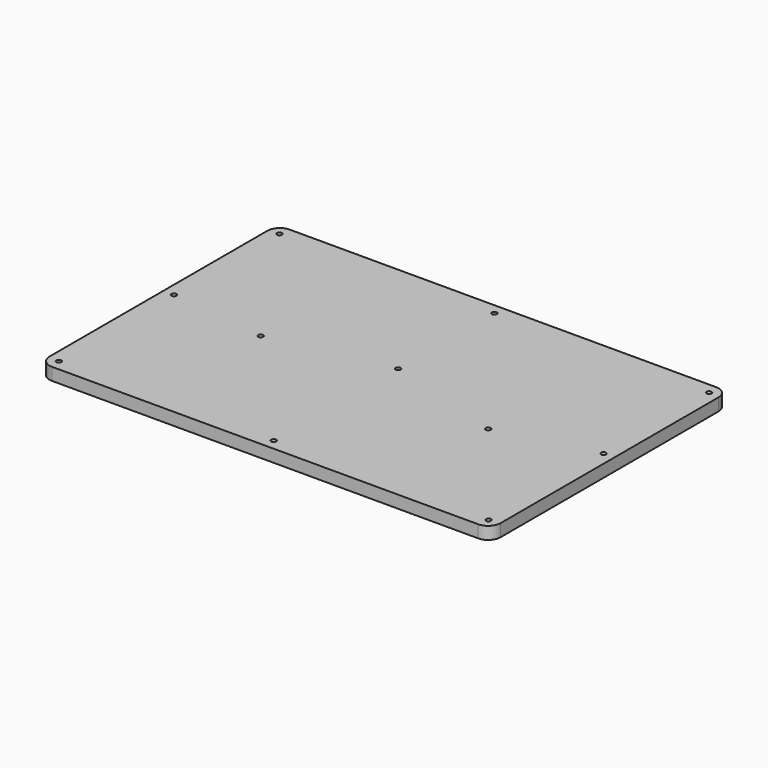
from build123d import *

# Parameters (mm, degrees)
F0_W     = 181.450293
F0_H     = 119.538183
F0_W_2   = 0.80067
F0_H_2   = 5.7989
F0_W_3   = 0.8006
F0_H_3   = 5.8003
F0_W_4   = 0.8007
F0_W_5   = 0.8008
F0_H_4   = 5.801
F0_H_5   = 5.8002
F0_H_6   = 5.7987
F0_W_6   = 0.801
F0_W_7   = 0.8
F0_W_8   = 0.875
F0_H_7   = 2.8002
F1_DEPTH = 5
F3_R     = 5
F2_R     = 1
F4_DEPTH = 5
F5_R     = 1.8
F5_R_2   = 1
F6_DEPTH = 2.5


# Not quite as in the source:
# - a feature names something its author has since deleted; it is built from what else it names


with BuildPart() as f1:
    # F0 (on Top) → F1 (new body)
    with BuildSketch(Plane.XY):
        with Locations((5e-07, 5e-07)):
            Rectangle(F0_W, F0_H)
        Polygon((-67.5631612539, -51.819168), (-73.900653, -51.819168), (-76.699453, -51.819168), (-85.1413756609, -51.819168), (-85.1413756609, -19.618408), (-76.699453, -19.618408), (-73.900653, -19.618408), (-67.5631612539, -19.618408), align=None, mode=Mode.SUBTRACT)
        Polygon((-49.349453, -43.381508), (-49.349453, -46.480608), (-49.349453, -48.281108), (-64.950353, -48.281108), (-64.950353, -46.480608), (-64.950353, -43.381508), (-64.950353, -37.581308), (-64.950353, -34.480708), (-64.950353, -32.681608), (-49.349453, -32.681608), (-49.349453, -34.480708), (-49.349453, -37.581308), align=None, mode=Mode.SUBTRACT)
        Polygon((-30.299453, -33.856508), (-30.299453, -36.955608), (-30.299453, -38.756108), (-45.900353, -38.756108), (-45.900353, -36.955608), (-45.900353, -33.856508), (-45.900353, -28.056308), (-45.900353, -24.955708), (-45.900353, -23.156508), (-30.299453, -23.156508), (-30.299453, -24.955708), (-30.299453, -28.056308), align=None, mode=Mode.SUBTRACT)
        Polygon((-11.249453, -38.619008), (-11.249453, -41.719508), (-11.249453, -43.518608), (-26.850353, -43.518608), (-26.850353, -41.719508), (-26.850353, -38.619008), (-26.850353, -32.818808), (-26.850353, -29.719608), (-26.850353, -27.919108), (-11.249453, -27.919108), (-11.249453, -29.719608), (-11.249453, -32.818808), align=None, mode=Mode.SUBTRACT)
        Polygon((-49.349453, -24.331508), (-49.349453, -27.430608), (-49.349453, -29.231108), (-64.950353, -29.231108), (-64.950353, -27.430608), (-64.950353, -24.331508), (-64.950353, -18.531208), (-64.950353, -15.430608), (-64.950353, -13.631508), (-49.349453, -13.631508), (-49.349453, -15.430608), (-49.349453, -18.531208), align=None, mode=Mode.SUBTRACT)
        Polygon((-68.399553, -10.044008), (-68.399553, -13.144608), (-68.399553, -14.943708), (-84.000333, -14.943708), (-84.000333, -13.144608), (-84.000333, -10.044008), (-84.000333, -4.243708), (-84.000333, -1.144508), (-84.000333, 0.655992), (-68.399553, 0.655992), (-68.399553, -1.144508), (-68.399553, -4.243708), align=None, mode=Mode.SUBTRACT)
        Polygon((-49.349453, -5.281508), (-49.349453, -8.380708), (-49.349453, -10.181208), (-64.950353, -10.181208), (-64.950353, -8.380708), (-64.950353, -5.281508), (-64.950353, 0.518792), (-64.950353, 3.619392), (-64.950353, 5.418492), (-49.349453, 5.418492), (-49.349453, 3.619392), (-49.349453, 0.518792), align=None, mode=Mode.SUBTRACT)
        Polygon((-11.249453, -19.569008), (-11.249453, -22.669608), (-11.249453, -24.468708), (-26.850353, -24.468708), (-26.850353, -22.669608), (-26.850353, -19.569008), (-26.850353, -13.768708), (-26.850353, -10.669508), (-26.850353, -8.869008), (-11.249453, -8.869008), (-11.249453, -10.669508), (-11.249453, -13.768708), align=None, mode=Mode.SUBTRACT)
        Polygon((-30.299453, -14.806508), (-30.299453, -17.905708), (-30.299453, -19.706208), (-45.900353, -19.706208), (-45.900353, -17.905708), (-45.900353, -14.806508), (-45.900353, -9.006208), (-45.900353, -5.905608), (-45.900353, -4.106508), (-30.299453, -4.106508), (-30.299453, -5.905608), (-30.299453, -9.006208), align=None, mode=Mode.SUBTRACT)
        Polygon((26.850147, -48.144008), (26.850147, -51.244528), (26.850147, -53.043638), (11.249147, -53.043638), (11.249147, -51.244528), (11.249147, -48.144008), (11.249147, -42.343808), (11.249147, -39.244608), (11.249147, -37.444108), (26.850147, -37.444108), (26.850147, -39.244608), (26.850147, -42.343808), align=None, mode=Mode.SUBTRACT)
        Polygon((45.900147, -48.144008), (45.900147, -51.244528), (45.900147, -53.043638), (30.299147, -53.043638), (30.299147, -51.244528), (30.299147, -48.144008), (30.299147, -42.343808), (30.299147, -39.244608), (30.299147, -37.444108), (45.900147, -37.444108), (45.900147, -39.244608), (45.900147, -42.343808), align=None, mode=Mode.SUBTRACT)
        Polygon((7.800547, -43.381508), (7.800547, -46.480608), (7.800547, -48.281108), (-7.800353, -48.281108), (-7.800353, -46.480608), (-7.800353, -43.381508), (-7.800353, -37.581308), (-7.800353, -34.480708), (-7.800353, -32.681608), (7.800547, -32.681608), (7.800547, -34.480708), (7.800547, -37.581308), align=None, mode=Mode.SUBTRACT)
        Polygon((82.775147, -45.744808), (81.900147, -45.744808), (81.900147, -52.014858), (81.900147, -54.3472580612), (50.575147, -54.3472580612), (50.575147, -45.744808), (50.575147, -42.944608), (50.575147, -37.444108), (81.900147, -37.444108), (81.900147, -39.714508), (81.900147, -42.944608), (82.775147, -42.944608), align=None, mode=Mode.SUBTRACT)
        Polygon((26.850147, -29.094008), (26.850147, -32.194508), (26.850147, -33.993608), (11.249147, -33.993608), (11.249147, -32.194508), (11.249147, -29.094008), (11.249147, -23.293708), (11.249147, -20.194508), (11.249147, -18.394008), (26.850147, -18.394008), (26.850147, -20.194508), (26.850147, -23.293708), align=None, mode=Mode.SUBTRACT)
        Polygon((7.800547, -24.331508), (7.800547, -27.430608), (7.800547, -29.571082443), (-7.800353, -29.571082443), (-7.800353, -27.430608), (-7.800353, -24.331508), (-7.800353, -18.531208), (-7.800353, -15.430608), (-7.800353, -13.4431961924), (7.800547, -13.4431961924), (7.800547, -15.430608), (7.800547, -18.531208), align=None, mode=Mode.SUBTRACT)
        Polygon((45.900147, -29.094008), (45.900147, -32.194508), (45.900147, -33.993608), (30.299147, -33.993608), (30.299147, -32.194508), (30.299147, -29.094008), (30.299147, -23.293708), (30.299147, -20.194508), (30.299147, -18.394008), (45.900147, -18.394008), (45.900147, -20.194508), (45.900147, -23.293708), align=None, mode=Mode.SUBTRACT)
        Polygon((7.800547, -5.281508), (7.800547, -8.380708), (7.800547, -10.181208), (-7.800353, -10.181208), (-7.800353, -8.380708), (-7.800353, -5.281508), (-7.800353, 0.518792), (-7.800353, 3.619392), (-7.800353, 5.418492), (7.800547, 5.418492), (7.800547, 3.619392), (7.800547, 0.518792), align=None, mode=Mode.SUBTRACT)
        Polygon((26.850147, -10.044008), (26.850147, -13.144608), (26.850147, -14.943708), (11.249147, -14.943708), (11.249147, -13.144608), (11.249147, -10.044008), (11.249147, -4.243708), (11.249147, -1.144508), (11.249147, 0.655992), (26.850147, 0.655992), (26.850147, -1.144508), (26.850147, -4.243708), align=None, mode=Mode.SUBTRACT)
        Polygon((45.900147, -10.044008), (45.900147, -13.144608), (45.900147, -14.943708), (30.299147, -14.943708), (30.299147, -13.144608), (30.299147, -10.044008), (30.299147, -4.243708), (30.299147, -1.144508), (30.299147, 0.655992), (45.900147, 0.655992), (45.900147, -1.144508), (45.900147, -4.243708), align=None, mode=Mode.SUBTRACT)
        Polygon((64.950147, -29.094008), (64.950147, -32.194508), (64.950147, -33.993608), (49.349147, -33.993608), (49.349147, -32.194508), (49.349147, -29.094008), (49.349147, -23.293708), (49.349147, -20.194508), (49.349147, -18.394008), (64.950147, -18.394008), (64.950147, -20.194508), (64.950147, -23.293708), align=None, mode=Mode.SUBTRACT)
        Polygon((84.000147, -29.094008), (84.000147, -32.194508), (84.000147, -33.993608), (68.399147, -33.993608), (68.399147, -32.194508), (68.399147, -29.094008), (68.399147, -23.293708), (68.399147, -20.194508), (68.399147, -18.394008), (84.000147, -18.394008), (84.000147, -20.194508), (84.000147, -23.293708), align=None, mode=Mode.SUBTRACT)
        Polygon((64.950147, -10.044008), (64.950147, -13.144608), (64.950147, -14.943708), (49.349147, -14.943708), (49.349147, -13.144608), (49.349147, -10.044008), (49.349147, -4.243708), (49.349147, -1.144508), (49.349147, 0.655992), (64.950147, 0.655992), (64.950147, -1.144508), (64.950147, -4.243708), align=None, mode=Mode.SUBTRACT)
        Polygon((84.000147, -10.044008), (84.000147, -13.144608), (84.000147, -14.943708), (68.399147, -14.943708), (68.399147, -13.144608), (68.399147, -10.044008), (68.399147, -4.243708), (68.399147, -1.144508), (68.399147, 0.655992), (84.000147, 0.655992), (84.000147, -1.144508), (84.000147, -4.243708), align=None, mode=Mode.SUBTRACT)
        Polygon((-68.399553, 9.005992), (-68.399553, 5.905392), (-68.399553, 4.106292), (-84.000333, 4.106292), (-84.000333, 5.905392), (-84.000333, 9.005992), (-84.000333, 14.806292), (-84.000333, 17.905492), (-84.000333, 19.705992), (-68.399553, 19.705992), (-68.399553, 17.905492), (-68.399553, 14.806292), align=None, mode=Mode.SUBTRACT)
        Polygon((-49.349453, 13.768492), (-49.349453, 10.669292), (-49.349453, 8.868792), (-64.950353, 8.868792), (-64.950353, 10.669292), (-64.950353, 13.768492), (-64.950353, 19.568792), (-64.950353, 22.669392), (-64.950353, 24.468492), (-49.349453, 24.468492), (-49.349453, 22.669392), (-49.349453, 19.568792), align=None, mode=Mode.SUBTRACT)
        Polygon((-30.299453, 4.243492), (-30.299453, 1.144292), (-30.299453, -0.656208), (-45.900353, -0.656208), (-45.900353, 1.144292), (-45.900353, 4.243492), (-45.900353, 10.043792), (-45.900353, 13.144392), (-45.900353, 14.943492), (-30.299453, 14.943492), (-30.299453, 13.144392), (-30.299453, 10.043792), align=None, mode=Mode.SUBTRACT)
        Polygon((-11.249453, -0.519008), (-11.249453, -3.619608), (-11.249453, -5.418708), (-26.850353, -5.418708), (-26.850353, -3.619608), (-26.850353, -0.519008), (-26.850353, 5.281292), (-26.850353, 8.380492), (-26.850353, 10.180992), (-11.249453, 10.180992), (-11.249453, 8.380492), (-11.249453, 5.281292), align=None, mode=Mode.SUBTRACT)
        Polygon((-30.299453, 23.293492), (-30.299453, 20.194292), (-30.299453, 17.9319474846), (-45.900353, 17.9319474846), (-45.900353, 20.194292), (-45.900353, 23.293492), (-45.900353, 29.093792), (-45.900353, 32.194392), (-45.900353, 33.993492), (-30.299453, 33.993492), (-30.299453, 32.194392), (-30.299453, 29.093792), align=None, mode=Mode.SUBTRACT)
        Polygon((-11.249453, 18.530992), (-11.249453, 15.430392), (-11.249453, 13.631292), (-26.850353, 13.631292), (-26.850353, 15.430392), (-26.850353, 18.530992), (-26.850353, 24.331292), (-26.850353, 27.430492), (-26.850353, 29.230992), (-11.249453, 29.230992), (-11.249453, 27.430492), (-11.249453, 24.331292), align=None, mode=Mode.SUBTRACT)
        Polygon((-68.399553, 28.057392), (-68.399553, 24.956792), (-68.399553, 23.156292), (-84.000333, 23.156292), (-84.000333, 24.956792), (-84.000333, 28.057392), (-84.000333, 33.856292), (-84.000333, 36.956892), (-84.000333, 38.757392), (-68.399553, 38.757392), (-68.399553, 36.956892), (-68.399553, 33.856292), align=None, mode=Mode.SUBTRACT)
        Polygon((-49.349453, 32.818492), (-49.349453, 29.719292), (-49.349453, 27.918792), (-64.950353, 27.918792), (-64.950353, 29.719292), (-64.950353, 32.818492), (-64.950353, 38.618792), (-64.950353, 41.719092), (-64.950353, 43.518092), (-49.349453, 43.518092), (-49.349453, 41.719092), (-49.349453, 38.618792), align=None, mode=Mode.SUBTRACT)
        Polygon((-11.249453, 37.582392), (-11.249453, 34.481792), (-11.249453, 32.681292), (-26.850353, 32.681292), (-26.850353, 34.481792), (-26.850353, 37.582392), (-26.850353, 43.381092), (-26.850353, 46.482092), (-26.850353, 48.282092), (-11.249453, 48.282092), (-11.249453, 46.482092), (-11.249453, 43.381092), align=None, mode=Mode.SUBTRACT)
        Polygon((-30.299453, 42.343092), (-30.299453, 39.244292), (-30.299453, 37.443792), (-45.900353, 37.443792), (-45.900353, 39.244292), (-45.900353, 42.343092), (-45.900353, 48.144092), (-45.900353, 51.244092), (-45.900353, 53.043092), (-30.299453, 53.043092), (-30.299453, 51.244092), (-30.299453, 48.144092), align=None, mode=Mode.SUBTRACT)
        Polygon((26.850147, 9.005992), (26.850147, 5.905392), (26.850147, 4.106292), (11.249147, 4.106292), (11.249147, 5.905392), (11.249147, 9.005992), (11.249147, 14.806292), (11.249147, 17.905492), (11.249147, 19.705992), (26.850147, 19.705992), (26.850147, 17.905492), (26.850147, 14.806292), align=None, mode=Mode.SUBTRACT)
        Polygon((45.900147, 9.005992), (45.900147, 5.905392), (45.900147, 4.106292), (30.299147, 4.106292), (30.299147, 5.905392), (30.299147, 9.005992), (30.299147, 14.806292), (30.299147, 17.905492), (30.299147, 19.705992), (45.900147, 19.705992), (45.900147, 17.905492), (45.900147, 14.806292), align=None, mode=Mode.SUBTRACT)
        Polygon((7.800547, 13.768492), (7.800547, 10.669292), (7.800547, 8.868792), (-7.800353, 8.868792), (-7.800353, 10.669292), (-7.800353, 13.768492), (-7.800353, 19.568792), (-7.800353, 22.669392), (-7.800353, 24.468492), (7.800547, 24.468492), (7.800547, 22.669392), (7.800547, 19.568792), align=None, mode=Mode.SUBTRACT)
        Polygon((64.950147, 9.005992), (64.950147, 5.905392), (64.950147, 4.106292), (49.349147, 4.106292), (49.349147, 5.905392), (49.349147, 9.005992), (49.349147, 14.806292), (49.349147, 17.905492), (49.349147, 19.705992), (64.950147, 19.705992), (64.950147, 17.905492), (64.950147, 14.806292), align=None, mode=Mode.SUBTRACT)
        Polygon((84.000147, 9.005992), (84.000147, 5.905392), (84.000147, 4.106292), (68.399147, 4.106292), (68.399147, 5.905392), (68.399147, 9.005992), (68.399147, 14.806292), (68.399147, 17.905492), (68.399147, 19.705992), (84.000147, 19.705992), (84.000147, 17.905492), (84.000147, 14.806292), align=None, mode=Mode.SUBTRACT)
        Polygon((7.800547, 32.818492), (7.800547, 29.719292), (7.800547, 27.918792), (-7.800353, 27.918792), (-7.800353, 29.719292), (-7.800353, 32.818492), (-7.800353, 38.618792), (-7.800353, 41.719092), (-7.800353, 43.518092), (7.800547, 43.518092), (7.800547, 41.719092), (7.800547, 38.618792), align=None, mode=Mode.SUBTRACT)
        Polygon((26.850147, 28.057392), (26.850147, 24.956792), (26.850147, 23.156292), (11.249147, 23.156292), (11.249147, 24.956792), (11.249147, 28.057392), (11.249147, 33.856292), (11.249147, 36.956892), (11.249147, 38.757392), (26.850147, 38.757392), (26.850147, 36.956892), (26.850147, 33.856292), align=None, mode=Mode.SUBTRACT)
        Polygon((45.900147, 28.057392), (45.900147, 24.956792), (45.900147, 23.156292), (30.299147, 23.156292), (30.299147, 24.956792), (30.299147, 28.057392), (30.299147, 33.856292), (30.299147, 36.956892), (30.299147, 38.757392), (45.900147, 38.757392), (45.900147, 36.956892), (45.900147, 33.856292), align=None, mode=Mode.SUBTRACT)
        Polygon((64.950147, 28.057392), (64.950147, 24.956792), (64.950147, 23.156292), (49.349147, 23.156292), (49.349147, 24.956792), (49.349147, 28.057392), (49.349147, 33.856292), (49.349147, 36.956892), (49.349147, 38.757392), (64.950147, 38.757392), (64.950147, 36.956892), (64.950147, 33.856292), align=None, mode=Mode.SUBTRACT)
        Polygon((84.000147, 28.057392), (84.000147, 24.956792), (84.000147, 23.156292), (68.399147, 23.156292), (68.399147, 24.956792), (68.399147, 28.057392), (68.399147, 33.856292), (68.399147, 36.956892), (68.399147, 38.757392), (84.000147, 38.757392), (84.000147, 36.956892), (84.000147, 33.856292), align=None, mode=Mode.SUBTRACT)
        Polygon((-69.200153, 36.956892), (-68.399553, 36.956892), (-68.399553, 38.757392), (-84.000333, 38.757392), (-84.000333, 36.956892), (-83.199663, 36.956892), (-83.199663, 37.957392), (-69.200153, 37.957392), align=None)
        with Locations((-83.599998, 30.956842)):
            Rectangle(F0_W_2, F0_H_2)
        Polygon((-68.399553, 24.956792), (-69.200153, 24.956792), (-69.200153, 23.956292), (-83.199663, 23.956292), (-83.199663, 24.956792), (-84.000333, 24.956792), (-84.000333, 23.156292), (-68.399553, 23.156292), align=None)
        with Locations((-68.799853, 30.956842)):
            Rectangle(F0_W_3, F0_H_2)
        Polygon((-69.200153, 17.905492), (-68.399553, 17.905492), (-68.399553, 19.705992), (-84.000333, 19.705992), (-84.000333, 17.905492), (-83.199663, 17.905492), (-83.199663, 18.905992), (-69.200153, 18.905992), align=None)
        with Locations((-83.599998, 11.906142)):
            Rectangle(F0_W_2, F0_H_3)
        Polygon((-68.399553, 5.905392), (-69.200153, 5.905392), (-69.200153, 4.906292), (-83.199663, 4.906292), (-83.199663, 5.905392), (-84.000333, 5.905392), (-84.000333, 4.106292), (-68.399553, 4.106292), align=None)
        with Locations((-68.799853, 11.906142)):
            Rectangle(F0_W_3, F0_H_3)
        Polygon((-49.349453, 29.719292), (-50.150253, 29.719292), (-50.150253, 28.718792), (-64.149653, 28.718792), (-64.149653, 29.719292), (-64.950353, 29.719292), (-64.950353, 27.918792), (-49.349453, 27.918792), align=None)
        with Locations((-64.550003, 35.718642)):
            Rectangle(F0_W_4, F0_H_3)
        Polygon((-50.150253, 41.719092), (-49.349453, 41.719092), (-49.349453, 43.518092), (-64.950353, 43.518092), (-64.950353, 41.719092), (-64.149653, 41.719092), (-64.149653, 42.718092), (-50.150253, 42.718092), align=None)
        with Locations((-49.749853, 35.718642)):
            Rectangle(F0_W_5, F0_H_3)
        Polygon((-50.150253, 22.669392), (-49.349453, 22.669392), (-49.349453, 24.468492), (-64.950353, 24.468492), (-64.950353, 22.669392), (-64.149653, 22.669392), (-64.149653, 23.668492), (-50.150253, 23.668492), align=None)
        with Locations((-64.550003, 16.668642)):
            Rectangle(F0_W_4, F0_H_3)
        with Locations((-49.749853, 16.668642)):
            Rectangle(F0_W_5, F0_H_3)
        Polygon((-49.349453, 10.669292), (-50.150253, 10.669292), (-50.150253, 9.668792), (-64.149653, 9.668792), (-64.149653, 10.669292), (-64.950353, 10.669292), (-64.950353, 8.868792), (-49.349453, 8.868792), align=None)
        Polygon((-30.299453, 1.144292), (-31.100253, 1.144292), (-31.100253, 0.143792), (-45.099553, 0.143792), (-45.099553, 1.144292), (-45.900353, 1.144292), (-45.900353, -0.656208), (-30.299453, -0.656208), align=None)
        with Locations((-45.499953, 7.143642)):
            Rectangle(F0_W_5, F0_H_3)
        Polygon((-31.100253, 13.144392), (-30.299453, 13.144392), (-30.299453, 14.943492), (-45.900353, 14.943492), (-45.900353, 13.144392), (-45.099553, 13.144392), (-45.099553, 14.143492), (-31.100253, 14.143492), align=None)
        with Locations((-30.699853, 7.143642)):
            Rectangle(F0_W_5, F0_H_3)
        Polygon((-30.299453, 20.194292), (-31.100253, 20.194292), (-31.100253, 19.193792), (-45.099553, 19.193792), (-45.099553, 20.194292), (-45.900353, 20.194292), (-45.900353, 17.9319474846), (-30.299453, 17.9319474846), align=None)
        with Locations((-30.699853, 26.193642)):
            Rectangle(F0_W_5, F0_H_3)
        with Locations((-45.499953, 26.193642)):
            Rectangle(F0_W_5, F0_H_3)
        Polygon((-31.100253, 32.194392), (-30.299453, 32.194392), (-30.299453, 33.993492), (-45.900353, 33.993492), (-45.900353, 32.194392), (-45.099553, 32.194392), (-45.099553, 33.193492), (-31.100253, 33.193492), align=None)
        Polygon((-30.299453, 39.244292), (-31.100253, 39.244292), (-31.100253, 38.243792), (-45.099553, 38.243792), (-45.099553, 39.244292), (-45.900353, 39.244292), (-45.900353, 37.443792), (-30.299453, 37.443792), align=None)
        with Locations((-45.499953, 45.243592)):
            Rectangle(F0_W_5, F0_H_4)
        Polygon((-31.100253, 51.244092), (-30.299453, 51.244092), (-30.299453, 53.043092), (-45.900353, 53.043092), (-45.900353, 51.244092), (-45.099553, 51.244092), (-45.099553, 52.243092), (-31.100253, 52.243092), align=None)
        with Locations((-30.699853, 45.243592)):
            Rectangle(F0_W_5, F0_H_4)
        Polygon((-69.200153, -1.144508), (-68.399553, -1.144508), (-68.399553, 0.655992), (-84.000333, 0.655992), (-84.000333, -1.144508), (-83.199663, -1.144508), (-83.199663, -0.144008), (-69.200153, -0.144008), align=None)
        with Locations((-83.599998, -7.143858)):
            Rectangle(F0_W_2, F0_H_3)
        with Locations((-68.799853, -7.143858)):
            Rectangle(F0_W_3, F0_H_3)
        Polygon((-68.399553, -13.144608), (-69.200153, -13.144608), (-69.200153, -14.143708), (-83.199663, -14.143708), (-83.199663, -13.144608), (-84.000333, -13.144608), (-84.000333, -14.943708), (-68.399553, -14.943708), align=None)
        Polygon((-49.349453, -8.380708), (-50.150253, -8.380708), (-50.150253, -9.381208), (-64.149653, -9.381208), (-64.149653, -8.380708), (-64.950353, -8.380708), (-64.950353, -10.181208), (-49.349453, -10.181208), align=None)
        with Locations((-64.550003, -2.381358)):
            Rectangle(F0_W_4, F0_H_3)
        Polygon((-50.150253, 3.619392), (-49.349453, 3.619392), (-49.349453, 5.418492), (-64.950353, 5.418492), (-64.950353, 3.619392), (-64.149653, 3.619392), (-64.149653, 4.618492), (-50.150253, 4.618492), align=None)
        with Locations((-49.749853, -2.381358)):
            Rectangle(F0_W_5, F0_H_3)
        Polygon((-69.200153, -42.718608), (-70.200653, -42.718608), (-70.200653, -43.519308), (-71.469853, -43.519308), (-71.469853, -44.293708), (-70.670553, -44.293708), (-70.670553, -46.019008), (-69.750053, -46.019008), (-69.750053, -49.319408), (-70.670553, -49.319408), (-70.670553, -50.944138), (-73.900653, -50.944138), (-73.900653, -51.819168), (-67.5631612539, -51.819168), (-67.5631612539, -19.618408), (-73.900653, -19.618408), (-73.900653, -20.493708), (-70.670553, -20.493708), (-70.670553, -22.119608), (-69.750053, -22.119608), (-69.750053, -25.418708), (-70.670553, -25.418708), (-70.670553, -27.144008), (-71.469853, -27.144008), (-71.469853, -27.919908), (-70.200653, -27.919908), (-70.200653, -28.719108), (-69.200153, -28.719108), align=None)
        Polygon((-85.1413756609, -51.819168), (-76.699453, -51.819168), (-76.699453, -50.944138), (-82.969543, -50.944138), (-82.969543, -49.319408), (-83.950693, -49.319408), (-83.950693, -46.019008), (-82.969543, -46.019008), (-82.969543, -44.293708), (-82.170293, -44.293708), (-82.170293, -43.519308), (-82.200593, -43.519308), (-82.200593, -42.718608), (-83.199663, -42.718608), (-83.199663, -28.719108), (-82.200593, -28.719108), (-82.200593, -27.919908), (-82.170293, -27.919908), (-82.170293, -27.144008), (-82.969543, -27.144008), (-82.969543, -25.418708), (-83.950693, -25.418708), (-83.950693, -22.119608), (-82.969543, -22.119608), (-82.969543, -20.493708), (-76.699453, -20.493708), (-76.699453, -19.618408), (-85.1413756609, -19.618408), align=None)
        Polygon((-49.349453, -27.430608), (-50.150253, -27.430608), (-50.150253, -28.431108), (-64.149653, -28.431108), (-64.149653, -27.430608), (-64.950353, -27.430608), (-64.950353, -29.231108), (-49.349453, -29.231108), align=None)
        with Locations((-64.550003, -21.431358)):
            Rectangle(F0_W_4, F0_H_3)
        Polygon((-50.150253, -15.430608), (-49.349453, -15.430608), (-49.349453, -13.631508), (-64.950353, -13.631508), (-64.950353, -15.430608), (-64.149653, -15.430608), (-64.149653, -14.431508), (-50.150253, -14.431508), align=None)
        with Locations((-49.749853, -21.431358)):
            Rectangle(F0_W_5, F0_H_3)
        Polygon((-50.150253, -34.480708), (-49.349453, -34.480708), (-49.349453, -32.681608), (-64.950353, -32.681608), (-64.950353, -34.480708), (-64.149653, -34.480708), (-64.149653, -33.481608), (-50.150253, -33.481608), align=None)
        with Locations((-49.749853, -40.481408)):
            Rectangle(F0_W_5, F0_H_5)
        with Locations((-64.550003, -40.481408)):
            Rectangle(F0_W_4, F0_H_5)
        Polygon((-49.349453, -46.480608), (-50.150253, -46.480608), (-50.150253, -47.481108), (-64.149653, -47.481108), (-64.149653, -46.480608), (-64.950353, -46.480608), (-64.950353, -48.281108), (-49.349453, -48.281108), align=None)
        Polygon((-30.299453, -36.955608), (-31.100253, -36.955608), (-31.100253, -37.956108), (-45.099553, -37.956108), (-45.099553, -36.955608), (-45.900353, -36.955608), (-45.900353, -38.756108), (-30.299453, -38.756108), align=None)
        with Locations((-30.699853, -30.956408)):
            Rectangle(F0_W_5, F0_H_5)
        with Locations((-45.499953, -30.956408)):
            Rectangle(F0_W_5, F0_H_5)
        Polygon((-31.100253, -24.955708), (-30.299453, -24.955708), (-30.299453, -23.156508), (-45.900353, -23.156508), (-45.900353, -24.955708), (-45.099553, -24.955708), (-45.099553, -23.956508), (-31.100253, -23.956508), align=None)
        Polygon((-30.299453, -17.905708), (-31.100253, -17.905708), (-31.100253, -18.906208), (-45.099553, -18.906208), (-45.099553, -17.905708), (-45.900353, -17.905708), (-45.900353, -19.706208), (-30.299453, -19.706208), align=None)
        with Locations((-45.499953, -11.906358)):
            Rectangle(F0_W_5, F0_H_3)
        Polygon((-31.100253, -5.905608), (-30.299453, -5.905608), (-30.299453, -4.106508), (-45.900353, -4.106508), (-45.900353, -5.905608), (-45.099553, -5.905608), (-45.099553, -4.906508), (-31.100253, -4.906508), align=None)
        with Locations((-30.699853, -11.906358)):
            Rectangle(F0_W_5, F0_H_3)
        Polygon((-11.249453, -41.719508), (-12.050253, -41.719508), (-12.050253, -42.718608), (-26.049553, -42.718608), (-26.049553, -41.719508), (-26.850353, -41.719508), (-26.850353, -43.518608), (-11.249453, -43.518608), align=None)
        with Locations((-26.449953, -35.718908)):
            Rectangle(F0_W_5, F0_H_5)
        Polygon((-12.050253, -29.719608), (-11.249453, -29.719608), (-11.249453, -27.919108), (-26.850353, -27.919108), (-26.850353, -29.719608), (-26.049553, -29.719608), (-26.049553, -28.719108), (-12.050253, -28.719108), align=None)
        with Locations((-11.649853, -35.718908)):
            Rectangle(F0_W_5, F0_H_5)
        Polygon((-11.249453, -22.669608), (-12.050253, -22.669608), (-12.050253, -23.668708), (-26.049553, -23.668708), (-26.049553, -22.669608), (-26.850353, -22.669608), (-26.850353, -24.468708), (-11.249453, -24.468708), align=None)
        with Locations((-11.649853, -16.668858)):
            Rectangle(F0_W_5, F0_H_3)
        with Locations((-26.449953, -16.668858)):
            Rectangle(F0_W_5, F0_H_3)
        Polygon((-12.050253, -10.669508), (-11.249453, -10.669508), (-11.249453, -8.869008), (-26.850353, -8.869008), (-26.850353, -10.669508), (-26.049553, -10.669508), (-26.049553, -9.669008), (-12.050253, -9.669008), align=None)
        Polygon((7.800547, -46.480608), (6.999747, -46.480608), (6.999747, -47.481108), (-6.999553, -47.481108), (-6.999553, -46.480608), (-7.800353, -46.480608), (-7.800353, -48.281108), (7.800547, -48.281108), align=None)
        with Locations((7.400147, -40.481408)):
            Rectangle(F0_W_5, F0_H_5)
        with Locations((-7.399953, -40.481408)):
            Rectangle(F0_W_5, F0_H_5)
        Polygon((6.999747, -34.480708), (7.800547, -34.480708), (7.800547, -32.681608), (-7.800353, -32.681608), (-7.800353, -34.480708), (-6.999553, -34.480708), (-6.999553, -33.481608), (6.999747, -33.481608), align=None)
        Polygon((7.800547, -27.430608), (6.999747, -27.430608), (6.999747, -28.431108), (-6.999553, -28.431108), (-6.999553, -27.430608), (-7.800353, -27.430608), (-7.800353, -29.571082443), (7.800547, -29.571082443), align=None)
        with Locations((-7.399953, -21.431358)):
            Rectangle(F0_W_5, F0_H_3)
        with Locations((7.400147, -21.431358)):
            Rectangle(F0_W_5, F0_H_3)
        Polygon((6.999747, -15.430608), (7.800547, -15.430608), (7.800547, -13.4431961924), (-7.800353, -13.4431961924), (-7.800353, -15.430608), (-6.999553, -15.430608), (-6.999553, -14.431508), (6.999747, -14.431508), align=None)
        Polygon((7.800547, -8.380708), (6.999747, -8.380708), (6.999747, -9.381208), (-6.999553, -9.381208), (-6.999553, -8.380708), (-7.800353, -8.380708), (-7.800353, -10.181208), (7.800547, -10.181208), align=None)
        with Locations((7.400147, -2.381358)):
            Rectangle(F0_W_5, F0_H_3)
        with Locations((-7.399953, -2.381358)):
            Rectangle(F0_W_5, F0_H_3)
        Polygon((6.999747, 3.619392), (7.800547, 3.619392), (7.800547, 5.418492), (-7.800353, 5.418492), (-7.800353, 3.619392), (-6.999553, 3.619392), (-6.999553, 4.618492), (6.999747, 4.618492), align=None)
        Polygon((-11.249453, -3.619608), (-12.050253, -3.619608), (-12.050253, -4.618708), (-26.049553, -4.618708), (-26.049553, -3.619608), (-26.850353, -3.619608), (-26.850353, -5.418708), (-11.249453, -5.418708), align=None)
        with Locations((-11.649853, 2.381142)):
            Rectangle(F0_W_5, F0_H_3)
        with Locations((-26.449953, 2.381142)):
            Rectangle(F0_W_5, F0_H_3)
        Polygon((-12.050253, 8.380492), (-11.249453, 8.380492), (-11.249453, 10.180992), (-26.850353, 10.180992), (-26.850353, 8.380492), (-26.049553, 8.380492), (-26.049553, 9.380992), (-12.050253, 9.380992), align=None)
        Polygon((-11.249453, 15.430392), (-12.050253, 15.430392), (-12.050253, 14.431292), (-26.049553, 14.431292), (-26.049553, 15.430392), (-26.850353, 15.430392), (-26.850353, 13.631292), (-11.249453, 13.631292), align=None)
        with Locations((-26.449953, 21.431142)):
            Rectangle(F0_W_5, F0_H_3)
        Polygon((-12.050253, 27.430492), (-11.249453, 27.430492), (-11.249453, 29.230992), (-26.850353, 29.230992), (-26.850353, 27.430492), (-26.049553, 27.430492), (-26.049553, 28.430992), (-12.050253, 28.430992), align=None)
        with Locations((-11.649853, 21.431142)):
            Rectangle(F0_W_5, F0_H_3)
        Polygon((7.800547, 10.669292), (6.999747, 10.669292), (6.999747, 9.668792), (-6.999553, 9.668792), (-6.999553, 10.669292), (-7.800353, 10.669292), (-7.800353, 8.868792), (7.800547, 8.868792), align=None)
        with Locations((-7.399953, 16.668642)):
            Rectangle(F0_W_5, F0_H_3)
        with Locations((7.400147, 16.668642)):
            Rectangle(F0_W_5, F0_H_3)
        Polygon((6.999747, 22.669392), (7.800547, 22.669392), (7.800547, 24.468492), (-7.800353, 24.468492), (-7.800353, 22.669392), (-6.999553, 22.669392), (-6.999553, 23.668492), (6.999747, 23.668492), align=None)
        Polygon((7.800547, 29.719292), (6.999747, 29.719292), (6.999747, 28.718792), (-6.999553, 28.718792), (-6.999553, 29.719292), (-7.800353, 29.719292), (-7.800353, 27.918792), (7.800547, 27.918792), align=None)
        with Locations((7.400147, 35.718642)):
            Rectangle(F0_W_5, F0_H_3)
        with Locations((-7.399953, 35.718642)):
            Rectangle(F0_W_5, F0_H_3)
        Polygon((6.999747, 41.719092), (7.800547, 41.719092), (7.800547, 43.518092), (-7.800353, 43.518092), (-7.800353, 41.719092), (-6.999553, 41.719092), (-6.999553, 42.718092), (6.999747, 42.718092), align=None)
        Polygon((-12.050253, 46.482092), (-11.249453, 46.482092), (-11.249453, 48.282092), (-26.850353, 48.282092), (-26.850353, 46.482092), (-26.049553, 46.482092), (-26.049553, 47.482092), (-12.050253, 47.482092), align=None)
        with Locations((-11.649853, 40.481742)):
            Rectangle(F0_W_5, F0_H_6)
        with Locations((-26.449953, 40.481742)):
            Rectangle(F0_W_5, F0_H_6)
        Polygon((-11.249453, 34.481792), (-12.050253, 34.481792), (-12.050253, 33.481292), (-26.049553, 33.481292), (-26.049553, 34.481792), (-26.850353, 34.481792), (-26.850353, 32.681292), (-11.249453, 32.681292), align=None)
        Polygon((26.050147, 36.956892), (26.850147, 36.956892), (26.850147, 38.757392), (11.249147, 38.757392), (11.249147, 36.956892), (12.050147, 36.956892), (12.050147, 37.957392), (26.050147, 37.957392), align=None)
        with Locations((11.649647, 30.956842)):
            Rectangle(F0_W_6, F0_H_2)
        Polygon((26.850147, 24.956792), (26.050147, 24.956792), (26.050147, 23.956292), (12.050147, 23.956292), (12.050147, 24.956792), (11.249147, 24.956792), (11.249147, 23.156292), (26.850147, 23.156292), align=None)
        with Locations((26.450147, 30.956842)):
            Rectangle(F0_W_7, F0_H_2)
        with Locations((30.699647, 30.956842)):
            Rectangle(F0_W_6, F0_H_2)
        Polygon((45.100147, 36.956892), (45.900147, 36.956892), (45.900147, 38.757392), (30.299147, 38.757392), (30.299147, 36.956892), (31.100147, 36.956892), (31.100147, 37.957392), (45.100147, 37.957392), align=None)
        with Locations((45.500147, 30.956842)):
            Rectangle(F0_W_7, F0_H_2)
        Polygon((45.900147, 24.956792), (45.100147, 24.956792), (45.100147, 23.956292), (31.100147, 23.956292), (31.100147, 24.956792), (30.299147, 24.956792), (30.299147, 23.156292), (45.900147, 23.156292), align=None)
        Polygon((64.950147, 24.956792), (64.150147, 24.956792), (64.150147, 23.956292), (50.150147, 23.956292), (50.150147, 24.956792), (49.349147, 24.956792), (49.349147, 23.156292), (64.950147, 23.156292), align=None)
        with Locations((49.749647, 30.956842)):
            Rectangle(F0_W_6, F0_H_2)
        Polygon((64.150147, 36.956892), (64.950147, 36.956892), (64.950147, 38.757392), (49.349147, 38.757392), (49.349147, 36.956892), (50.150147, 36.956892), (50.150147, 37.957392), (64.150147, 37.957392), align=None)
        with Locations((64.550147, 30.956842)):
            Rectangle(F0_W_7, F0_H_2)
        with Locations((68.799647, 30.956842)):
            Rectangle(F0_W_6, F0_H_2)
        Polygon((83.200147, 36.956892), (84.000147, 36.956892), (84.000147, 38.757392), (68.399147, 38.757392), (68.399147, 36.956892), (69.200147, 36.956892), (69.200147, 37.957392), (83.200147, 37.957392), align=None)
        with Locations((83.600147, 30.956842)):
            Rectangle(F0_W_7, F0_H_2)
        Polygon((84.000147, 24.956792), (83.200147, 24.956792), (83.200147, 23.956292), (69.200147, 23.956292), (69.200147, 24.956792), (68.399147, 24.956792), (68.399147, 23.156292), (84.000147, 23.156292), align=None)
        Polygon((83.200147, 17.905492), (84.000147, 17.905492), (84.000147, 19.705992), (68.399147, 19.705992), (68.399147, 17.905492), (69.200147, 17.905492), (69.200147, 18.905992), (83.200147, 18.905992), align=None)
        with Locations((83.600147, 11.906142)):
            Rectangle(F0_W_7, F0_H_3)
        Polygon((84.000147, 5.905392), (83.200147, 5.905392), (83.200147, 4.906292), (69.200147, 4.906292), (69.200147, 5.905392), (68.399147, 5.905392), (68.399147, 4.106292), (84.000147, 4.106292), align=None)
        with Locations((68.799647, 11.906142)):
            Rectangle(F0_W_6, F0_H_3)
        Polygon((83.200147, -1.144508), (84.000147, -1.144508), (84.000147, 0.655992), (68.399147, 0.655992), (68.399147, -1.144508), (69.200147, -1.144508), (69.200147, -0.144008), (83.200147, -0.144008), align=None)
        with Locations((68.799647, -7.143858)):
            Rectangle(F0_W_6, F0_H_3)
        Polygon((84.000147, -13.144608), (83.200147, -13.144608), (83.200147, -14.143708), (69.200147, -14.143708), (69.200147, -13.144608), (68.399147, -13.144608), (68.399147, -14.943708), (84.000147, -14.943708), align=None)
        with Locations((83.600147, -7.143858)):
            Rectangle(F0_W_7, F0_H_3)
        with Locations((64.550147, 11.906142)):
            Rectangle(F0_W_7, F0_H_3)
        Polygon((64.150147, 17.905492), (64.950147, 17.905492), (64.950147, 19.705992), (49.349147, 19.705992), (49.349147, 17.905492), (50.150147, 17.905492), (50.150147, 18.905992), (64.150147, 18.905992), align=None)
        with Locations((49.749647, 11.906142)):
            Rectangle(F0_W_6, F0_H_3)
        Polygon((64.950147, 5.905392), (64.150147, 5.905392), (64.150147, 4.906292), (50.150147, 4.906292), (50.150147, 5.905392), (49.349147, 5.905392), (49.349147, 4.106292), (64.950147, 4.106292), align=None)
        Polygon((64.150147, -1.144508), (64.950147, -1.144508), (64.950147, 0.655992), (49.349147, 0.655992), (49.349147, -1.144508), (50.150147, -1.144508), (50.150147, -0.144008), (64.150147, -0.144008), align=None)
        with Locations((49.749647, -7.143858)):
            Rectangle(F0_W_6, F0_H_3)
        Polygon((64.950147, -13.144608), (64.150147, -13.144608), (64.150147, -14.143708), (50.150147, -14.143708), (50.150147, -13.144608), (49.349147, -13.144608), (49.349147, -14.943708), (64.950147, -14.943708), align=None)
        with Locations((64.550147, -7.143858)):
            Rectangle(F0_W_7, F0_H_3)
        Polygon((45.100147, -1.144508), (45.900147, -1.144508), (45.900147, 0.655992), (30.299147, 0.655992), (30.299147, -1.144508), (31.100147, -1.144508), (31.100147, -0.144008), (45.100147, -0.144008), align=None)
        with Locations((45.500147, -7.143858)):
            Rectangle(F0_W_7, F0_H_3)
        with Locations((30.699647, -7.143858)):
            Rectangle(F0_W_6, F0_H_3)
        Polygon((45.900147, -13.144608), (45.100147, -13.144608), (45.100147, -14.143708), (31.100147, -14.143708), (31.100147, -13.144608), (30.299147, -13.144608), (30.299147, -14.943708), (45.900147, -14.943708), align=None)
        Polygon((45.900147, 5.905392), (45.100147, 5.905392), (45.100147, 4.906292), (31.100147, 4.906292), (31.100147, 5.905392), (30.299147, 5.905392), (30.299147, 4.106292), (45.900147, 4.106292), align=None)
        with Locations((30.699647, 11.906142)):
            Rectangle(F0_W_6, F0_H_3)
        Polygon((45.100147, 17.905492), (45.900147, 17.905492), (45.900147, 19.705992), (30.299147, 19.705992), (30.299147, 17.905492), (31.100147, 17.905492), (31.100147, 18.905992), (45.100147, 18.905992), align=None)
        with Locations((45.500147, 11.906142)):
            Rectangle(F0_W_7, F0_H_3)
        Polygon((26.050147, 17.905492), (26.850147, 17.905492), (26.850147, 19.705992), (11.249147, 19.705992), (11.249147, 17.905492), (12.050147, 17.905492), (12.050147, 18.905992), (26.050147, 18.905992), align=None)
        with Locations((11.649647, 11.906142)):
            Rectangle(F0_W_6, F0_H_3)
        Polygon((26.850147, 5.905392), (26.050147, 5.905392), (26.050147, 4.906292), (12.050147, 4.906292), (12.050147, 5.905392), (11.249147, 5.905392), (11.249147, 4.106292), (26.850147, 4.106292), align=None)
        with Locations((26.450147, 11.906142)):
            Rectangle(F0_W_7, F0_H_3)
        Polygon((26.050147, -1.144508), (26.850147, -1.144508), (26.850147, 0.655992), (11.249147, 0.655992), (11.249147, -1.144508), (12.050147, -1.144508), (12.050147, -0.144008), (26.050147, -0.144008), align=None)
        with Locations((11.649647, -7.143858)):
            Rectangle(F0_W_6, F0_H_3)
        Polygon((26.850147, -13.144608), (26.050147, -13.144608), (26.050147, -14.143708), (12.050147, -14.143708), (12.050147, -13.144608), (11.249147, -13.144608), (11.249147, -14.943708), (26.850147, -14.943708), align=None)
        with Locations((26.450147, -7.143858)):
            Rectangle(F0_W_7, F0_H_3)
        Polygon((26.050147, -20.194508), (26.850147, -20.194508), (26.850147, -18.394008), (11.249147, -18.394008), (11.249147, -20.194508), (12.050147, -20.194508), (12.050147, -19.194008), (26.050147, -19.194008), align=None)
        with Locations((26.450147, -26.193858)):
            Rectangle(F0_W_7, F0_H_3)
        with Locations((11.649647, -26.193858)):
            Rectangle(F0_W_6, F0_H_3)
        Polygon((26.850147, -32.194508), (26.050147, -32.194508), (26.050147, -33.193608), (12.050147, -33.193608), (12.050147, -32.194508), (11.249147, -32.194508), (11.249147, -33.993608), (26.850147, -33.993608), align=None)
        Polygon((26.050147, -39.244608), (26.850147, -39.244608), (26.850147, -37.444108), (11.249147, -37.444108), (11.249147, -39.244608), (12.050147, -39.244608), (12.050147, -38.244108), (26.050147, -38.244108), align=None)
        with Locations((11.649647, -45.243908)):
            Rectangle(F0_W_6, F0_H_5)
        Polygon((26.850147, -51.244528), (26.050147, -51.244528), (26.050147, -52.243638), (12.050147, -52.243638), (12.050147, -51.244528), (11.249147, -51.244528), (11.249147, -53.043638), (26.850147, -53.043638), align=None)
        with Locations((26.450147, -45.243908)):
            Rectangle(F0_W_7, F0_H_5)
        with Locations((30.699647, -45.243908)):
            Rectangle(F0_W_6, F0_H_5)
        Polygon((45.100147, -39.244608), (45.900147, -39.244608), (45.900147, -37.444108), (30.299147, -37.444108), (30.299147, -39.244608), (31.100147, -39.244608), (31.100147, -38.244108), (45.100147, -38.244108), align=None)
        Polygon((45.900147, -51.244528), (45.100147, -51.244528), (45.100147, -52.243638), (31.100147, -52.243638), (31.100147, -51.244528), (30.299147, -51.244528), (30.299147, -53.043638), (45.900147, -53.043638), align=None)
        with Locations((45.500147, -45.243908)):
            Rectangle(F0_W_7, F0_H_5)
        with Locations((45.500147, -26.193858)):
            Rectangle(F0_W_7, F0_H_3)
        Polygon((45.100147, -20.194508), (45.900147, -20.194508), (45.900147, -18.394008), (30.299147, -18.394008), (30.299147, -20.194508), (31.100147, -20.194508), (31.100147, -19.194008), (45.100147, -19.194008), align=None)
        with Locations((30.699647, -26.193858)):
            Rectangle(F0_W_6, F0_H_3)
        Polygon((45.900147, -32.194508), (45.100147, -32.194508), (45.100147, -33.193608), (31.100147, -33.193608), (31.100147, -32.194508), (30.299147, -32.194508), (30.299147, -33.993608), (45.900147, -33.993608), align=None)
        with Locations((49.749647, -26.193858)):
            Rectangle(F0_W_6, F0_H_3)
        Polygon((64.150147, -20.194508), (64.950147, -20.194508), (64.950147, -18.394008), (49.349147, -18.394008), (49.349147, -20.194508), (50.150147, -20.194508), (50.150147, -19.194008), (64.150147, -19.194008), align=None)
        with Locations((64.550147, -26.193858)):
            Rectangle(F0_W_7, F0_H_3)
        Polygon((64.950147, -32.194508), (64.150147, -32.194508), (64.150147, -33.193608), (50.150147, -33.193608), (50.150147, -32.194508), (49.349147, -32.194508), (49.349147, -33.993608), (64.950147, -33.993608), align=None)
        Polygon((80.274147, -39.714508), (81.900147, -39.714508), (81.900147, -37.444108), (50.575147, -37.444108), (50.575147, -42.944608), (51.450147, -42.944608), (51.450147, -39.714508), (53.074147, -39.714508), (53.074147, -38.794008), (56.375147, -38.794008), (56.375147, -39.714508), (58.100147, -39.714508), (58.100147, -40.513808), (58.874147, -40.513808), (58.874147, -39.244608), (59.675147, -39.244608), (59.675147, -38.244108), (73.675147, -38.244108), (73.675147, -39.244608), (74.475147, -39.244608), (74.475147, -40.513808), (75.250147, -40.513808), (75.250147, -39.714508), (76.975147, -39.714508), (76.975147, -38.794008), (80.274147, -38.794008), align=None)
        Polygon((81.900147, -54.3472580612), (81.900147, -52.014858), (80.274147, -52.014858), (80.274147, -52.994658), (76.975147, -52.994658), (76.975147, -52.014858), (75.250147, -52.014858), (75.250147, -51.214228), (74.475147, -51.214228), (74.475147, -51.244528), (73.675147, -51.244528), (73.675147, -52.243638), (59.675147, -52.243638), (59.675147, -51.244528), (58.874147, -51.244528), (58.874147, -51.214228), (58.100147, -51.214228), (58.100147, -52.014858), (56.375147, -52.014858), (56.375147, -52.994658), (53.074147, -52.994658), (53.074147, -52.014858), (51.450147, -52.014858), (51.450147, -45.744808), (50.575147, -45.744808), (50.575147, -54.3472580612), align=None)
        Polygon((83.200147, -20.194508), (84.000147, -20.194508), (84.000147, -18.394008), (68.399147, -18.394008), (68.399147, -20.194508), (69.200147, -20.194508), (69.200147, -19.194008), (83.200147, -19.194008), align=None)
        with Locations((83.600147, -26.193858)):
            Rectangle(F0_W_7, F0_H_3)
        with Locations((68.799647, -26.193858)):
            Rectangle(F0_W_6, F0_H_3)
        Polygon((84.000147, -32.194508), (83.200147, -32.194508), (83.200147, -33.193608), (69.200147, -33.193608), (69.200147, -32.194508), (68.399147, -32.194508), (68.399147, -33.993608), (84.000147, -33.993608), align=None)
        Polygon((-69.200153, 23.956292), (-69.200153, 24.956792), (-68.399553, 24.956792), (-68.399553, 28.057392), (-69.200153, 28.057392), (-69.200153, 33.856292), (-68.399553, 33.856292), (-68.399553, 36.956892), (-69.200153, 36.956892), (-69.200153, 37.957392), (-83.199663, 37.957392), (-83.199663, 36.956892), (-84.000333, 36.956892), (-84.000333, 33.856292), (-83.199663, 33.856292), (-83.199663, 28.057392), (-84.000333, 28.057392), (-84.000333, 24.956792), (-83.199663, 24.956792), (-83.199663, 23.956292), align=None)
        Polygon((-50.150253, 28.718792), (-50.150253, 29.719292), (-49.349453, 29.719292), (-49.349453, 32.818492), (-50.150253, 32.818492), (-50.150253, 38.618792), (-49.349453, 38.618792), (-49.349453, 41.719092), (-50.150253, 41.719092), (-50.150253, 42.718092), (-64.149653, 42.718092), (-64.149653, 41.719092), (-64.950353, 41.719092), (-64.950353, 38.618792), (-64.149653, 38.618792), (-64.149653, 32.818492), (-64.950353, 32.818492), (-64.950353, 29.719292), (-64.149653, 29.719292), (-64.149653, 28.718792), align=None)
        Polygon((-31.100253, 38.243792), (-31.100253, 39.244292), (-30.299453, 39.244292), (-30.299453, 42.343092), (-31.100253, 42.343092), (-31.100253, 48.144092), (-30.299453, 48.144092), (-30.299453, 51.244092), (-31.100253, 51.244092), (-31.100253, 52.243092), (-45.099553, 52.243092), (-45.099553, 51.244092), (-45.900353, 51.244092), (-45.900353, 48.144092), (-45.099553, 48.144092), (-45.099553, 42.343092), (-45.900353, 42.343092), (-45.900353, 39.244292), (-45.099553, 39.244292), (-45.099553, 38.243792), align=None)
        Polygon((-12.050253, 33.481292), (-12.050253, 34.481792), (-11.249453, 34.481792), (-11.249453, 37.582392), (-12.050253, 37.582392), (-12.050253, 43.381092), (-11.249453, 43.381092), (-11.249453, 46.482092), (-12.050253, 46.482092), (-12.050253, 47.482092), (-26.049553, 47.482092), (-26.049553, 46.482092), (-26.850353, 46.482092), (-26.850353, 43.381092), (-26.049553, 43.381092), (-26.049553, 37.582392), (-26.850353, 37.582392), (-26.850353, 34.481792), (-26.049553, 34.481792), (-26.049553, 33.481292), align=None)
        Polygon((6.999747, 28.718792), (6.999747, 29.719292), (7.800547, 29.719292), (7.800547, 32.818492), (6.999747, 32.818492), (6.999747, 38.618792), (7.800547, 38.618792), (7.800547, 41.719092), (6.999747, 41.719092), (6.999747, 42.718092), (-6.999553, 42.718092), (-6.999553, 41.719092), (-7.800353, 41.719092), (-7.800353, 38.618792), (-6.999553, 38.618792), (-6.999553, 32.818492), (-7.800353, 32.818492), (-7.800353, 29.719292), (-6.999553, 29.719292), (-6.999553, 28.718792), align=None)
        Polygon((6.999747, 9.668792), (6.999747, 10.669292), (7.800547, 10.669292), (7.800547, 13.768492), (6.999747, 13.768492), (6.999747, 19.568792), (7.800547, 19.568792), (7.800547, 22.669392), (6.999747, 22.669392), (6.999747, 23.668492), (-6.999553, 23.668492), (-6.999553, 22.669392), (-7.800353, 22.669392), (-7.800353, 19.568792), (-6.999553, 19.568792), (-6.999553, 13.768492), (-7.800353, 13.768492), (-7.800353, 10.669292), (-6.999553, 10.669292), (-6.999553, 9.668792), align=None)
        Polygon((-12.050253, 14.431292), (-12.050253, 15.430392), (-11.249453, 15.430392), (-11.249453, 18.530992), (-12.050253, 18.530992), (-12.050253, 24.331292), (-11.249453, 24.331292), (-11.249453, 27.430492), (-12.050253, 27.430492), (-12.050253, 28.430992), (-26.049553, 28.430992), (-26.049553, 27.430492), (-26.850353, 27.430492), (-26.850353, 24.331292), (-26.049553, 24.331292), (-26.049553, 18.530992), (-26.850353, 18.530992), (-26.850353, 15.430392), (-26.049553, 15.430392), (-26.049553, 14.431292), align=None)
        Polygon((-31.100253, 19.193792), (-31.100253, 20.194292), (-30.299453, 20.194292), (-30.299453, 23.293492), (-31.100253, 23.293492), (-31.100253, 29.093792), (-30.299453, 29.093792), (-30.299453, 32.194392), (-31.100253, 32.194392), (-31.100253, 33.193492), (-45.099553, 33.193492), (-45.099553, 32.194392), (-45.900353, 32.194392), (-45.900353, 29.093792), (-45.099553, 29.093792), (-45.099553, 23.293492), (-45.900353, 23.293492), (-45.900353, 20.194292), (-45.099553, 20.194292), (-45.099553, 19.193792), align=None)
        Polygon((-50.150253, 9.668792), (-50.150253, 10.669292), (-49.349453, 10.669292), (-49.349453, 13.768492), (-50.150253, 13.768492), (-50.150253, 19.568792), (-49.349453, 19.568792), (-49.349453, 22.669392), (-50.150253, 22.669392), (-50.150253, 23.668492), (-64.149653, 23.668492), (-64.149653, 22.669392), (-64.950353, 22.669392), (-64.950353, 19.568792), (-64.149653, 19.568792), (-64.149653, 13.768492), (-64.950353, 13.768492), (-64.950353, 10.669292), (-64.149653, 10.669292), (-64.149653, 9.668792), align=None)
        Polygon((-69.200153, 4.906292), (-69.200153, 5.905392), (-68.399553, 5.905392), (-68.399553, 9.005992), (-69.200153, 9.005992), (-69.200153, 14.806292), (-68.399553, 14.806292), (-68.399553, 17.905492), (-69.200153, 17.905492), (-69.200153, 18.905992), (-83.199663, 18.905992), (-83.199663, 17.905492), (-84.000333, 17.905492), (-84.000333, 14.806292), (-83.199663, 14.806292), (-83.199663, 9.005992), (-84.000333, 9.005992), (-84.000333, 5.905392), (-83.199663, 5.905392), (-83.199663, 4.906292), align=None)
        Polygon((-69.200153, -14.143708), (-69.200153, -13.144608), (-68.399553, -13.144608), (-68.399553, -10.044008), (-69.200153, -10.044008), (-69.200153, -4.243708), (-68.399553, -4.243708), (-68.399553, -1.144508), (-69.200153, -1.144508), (-69.200153, -0.144008), (-83.199663, -0.144008), (-83.199663, -1.144508), (-84.000333, -1.144508), (-84.000333, -4.243708), (-83.199663, -4.243708), (-83.199663, -10.044008), (-84.000333, -10.044008), (-84.000333, -13.144608), (-83.199663, -13.144608), (-83.199663, -14.143708), align=None)
        Polygon((-50.150253, -9.381208), (-50.150253, -8.380708), (-49.349453, -8.380708), (-49.349453, -5.281508), (-50.150253, -5.281508), (-50.150253, 0.518792), (-49.349453, 0.518792), (-49.349453, 3.619392), (-50.150253, 3.619392), (-50.150253, 4.618492), (-64.149653, 4.618492), (-64.149653, 3.619392), (-64.950353, 3.619392), (-64.950353, 0.518792), (-64.149653, 0.518792), (-64.149653, -5.281508), (-64.950353, -5.281508), (-64.950353, -8.380708), (-64.149653, -8.380708), (-64.149653, -9.381208), align=None)
        Polygon((-31.100253, 0.143792), (-31.100253, 1.144292), (-30.299453, 1.144292), (-30.299453, 4.243492), (-31.100253, 4.243492), (-31.100253, 10.043792), (-30.299453, 10.043792), (-30.299453, 13.144392), (-31.100253, 13.144392), (-31.100253, 14.143492), (-45.099553, 14.143492), (-45.099553, 13.144392), (-45.900353, 13.144392), (-45.900353, 10.043792), (-45.099553, 10.043792), (-45.099553, 4.243492), (-45.900353, 4.243492), (-45.900353, 1.144292), (-45.099553, 1.144292), (-45.099553, 0.143792), align=None)
        Polygon((-12.050253, -4.618708), (-12.050253, -3.619608), (-11.249453, -3.619608), (-11.249453, -0.519008), (-12.050253, -0.519008), (-12.050253, 5.281292), (-11.249453, 5.281292), (-11.249453, 8.380492), (-12.050253, 8.380492), (-12.050253, 9.380992), (-26.049553, 9.380992), (-26.049553, 8.380492), (-26.850353, 8.380492), (-26.850353, 5.281292), (-26.049553, 5.281292), (-26.049553, -0.519008), (-26.850353, -0.519008), (-26.850353, -3.619608), (-26.049553, -3.619608), (-26.049553, -4.618708), align=None)
        Polygon((6.999747, -9.381208), (6.999747, -8.380708), (7.800547, -8.380708), (7.800547, -5.281508), (6.999747, -5.281508), (6.999747, 0.518792), (7.800547, 0.518792), (7.800547, 3.619392), (6.999747, 3.619392), (6.999747, 4.618492), (-6.999553, 4.618492), (-6.999553, 3.619392), (-7.800353, 3.619392), (-7.800353, 0.518792), (-6.999553, 0.518792), (-6.999553, -5.281508), (-7.800353, -5.281508), (-7.800353, -8.380708), (-6.999553, -8.380708), (-6.999553, -9.381208), align=None)
        Polygon((6.999747, -28.431108), (6.999747, -27.430608), (7.800547, -27.430608), (7.800547, -24.331508), (6.999747, -24.331508), (6.999747, -18.531208), (7.800547, -18.531208), (7.800547, -15.430608), (6.999747, -15.430608), (6.999747, -14.431508), (-6.999553, -14.431508), (-6.999553, -15.430608), (-7.800353, -15.430608), (-7.800353, -18.531208), (-6.999553, -18.531208), (-6.999553, -24.331508), (-7.800353, -24.331508), (-7.800353, -27.430608), (-6.999553, -27.430608), (-6.999553, -28.431108), align=None)
        Polygon((-12.050253, -23.668708), (-12.050253, -22.669608), (-11.249453, -22.669608), (-11.249453, -19.569008), (-12.050253, -19.569008), (-12.050253, -13.768708), (-11.249453, -13.768708), (-11.249453, -10.669508), (-12.050253, -10.669508), (-12.050253, -9.669008), (-26.049553, -9.669008), (-26.049553, -10.669508), (-26.850353, -10.669508), (-26.850353, -13.768708), (-26.049553, -13.768708), (-26.049553, -19.569008), (-26.850353, -19.569008), (-26.850353, -22.669608), (-26.049553, -22.669608), (-26.049553, -23.668708), align=None)
        Polygon((-31.100253, -18.906208), (-31.100253, -17.905708), (-30.299453, -17.905708), (-30.299453, -14.806508), (-31.100253, -14.806508), (-31.100253, -9.006208), (-30.299453, -9.006208), (-30.299453, -5.905608), (-31.100253, -5.905608), (-31.100253, -4.906508), (-45.099553, -4.906508), (-45.099553, -5.905608), (-45.900353, -5.905608), (-45.900353, -9.006208), (-45.099553, -9.006208), (-45.099553, -14.806508), (-45.900353, -14.806508), (-45.900353, -17.905708), (-45.099553, -17.905708), (-45.099553, -18.906208), align=None)
        Polygon((-50.150253, -28.431108), (-50.150253, -27.430608), (-49.349453, -27.430608), (-49.349453, -24.331508), (-50.150253, -24.331508), (-50.150253, -18.531208), (-49.349453, -18.531208), (-49.349453, -15.430608), (-50.150253, -15.430608), (-50.150253, -14.431508), (-64.149653, -14.431508), (-64.149653, -15.430608), (-64.950353, -15.430608), (-64.950353, -18.531208), (-64.149653, -18.531208), (-64.149653, -24.331508), (-64.950353, -24.331508), (-64.950353, -27.430608), (-64.149653, -27.430608), (-64.149653, -28.431108), align=None)
        Polygon((-70.200653, -43.519308), (-70.200653, -42.718608), (-69.200153, -42.718608), (-69.200153, -28.719108), (-70.200653, -28.719108), (-70.200653, -27.919908), (-71.469853, -27.919908), (-71.469853, -27.144008), (-70.670553, -27.144008), (-70.670553, -25.418708), (-69.750053, -25.418708), (-69.750053, -22.119608), (-70.670553, -22.119608), (-70.670553, -20.493708), (-73.900653, -20.493708), (-73.900653, -19.618408), (-76.699453, -19.618408), (-76.699453, -20.493708), (-82.969543, -20.493708), (-82.969543, -22.119608), (-83.950693, -22.119608), (-83.950693, -25.418708), (-82.969543, -25.418708), (-82.969543, -27.144008), (-82.170293, -27.144008), (-82.170293, -27.919908), (-82.200593, -27.919908), (-82.200593, -28.719108), (-83.199663, -28.719108), (-83.199663, -42.718608), (-82.200593, -42.718608), (-82.200593, -43.519308), (-82.170293, -43.519308), (-82.170293, -44.293708), (-82.969543, -44.293708), (-82.969543, -46.019008), (-83.950693, -46.019008), (-83.950693, -49.319408), (-82.969543, -49.319408), (-82.969543, -50.944138), (-76.699453, -50.944138), (-76.699453, -51.819168), (-73.900653, -51.819168), (-73.900653, -50.944138), (-70.670553, -50.944138), (-70.670553, -49.319408), (-69.750053, -49.319408), (-69.750053, -46.019008), (-70.670553, -46.019008), (-70.670553, -44.293708), (-71.469853, -44.293708), (-71.469853, -43.519308), align=None)
        Polygon((-50.150253, -47.481108), (-50.150253, -46.480608), (-49.349453, -46.480608), (-49.349453, -43.381508), (-50.150253, -43.381508), (-50.150253, -37.581308), (-49.349453, -37.581308), (-49.349453, -34.480708), (-50.150253, -34.480708), (-50.150253, -33.481608), (-64.149653, -33.481608), (-64.149653, -34.480708), (-64.950353, -34.480708), (-64.950353, -37.581308), (-64.149653, -37.581308), (-64.149653, -43.381508), (-64.950353, -43.381508), (-64.950353, -46.480608), (-64.149653, -46.480608), (-64.149653, -47.481108), align=None)
        Polygon((-31.100253, -37.956108), (-31.100253, -36.955608), (-30.299453, -36.955608), (-30.299453, -33.856508), (-31.100253, -33.856508), (-31.100253, -28.056308), (-30.299453, -28.056308), (-30.299453, -24.955708), (-31.100253, -24.955708), (-31.100253, -23.956508), (-45.099553, -23.956508), (-45.099553, -24.955708), (-45.900353, -24.955708), (-45.900353, -28.056308), (-45.099553, -28.056308), (-45.099553, -33.856508), (-45.900353, -33.856508), (-45.900353, -36.955608), (-45.099553, -36.955608), (-45.099553, -37.956108), align=None)
        Polygon((-12.050253, -42.718608), (-12.050253, -41.719508), (-11.249453, -41.719508), (-11.249453, -38.619008), (-12.050253, -38.619008), (-12.050253, -32.818808), (-11.249453, -32.818808), (-11.249453, -29.719608), (-12.050253, -29.719608), (-12.050253, -28.719108), (-26.049553, -28.719108), (-26.049553, -29.719608), (-26.850353, -29.719608), (-26.850353, -32.818808), (-26.049553, -32.818808), (-26.049553, -38.619008), (-26.850353, -38.619008), (-26.850353, -41.719508), (-26.049553, -41.719508), (-26.049553, -42.718608), align=None)
        Polygon((6.999747, -47.481108), (6.999747, -46.480608), (7.800547, -46.480608), (7.800547, -43.381508), (6.999747, -43.381508), (6.999747, -37.581308), (7.800547, -37.581308), (7.800547, -34.480708), (6.999747, -34.480708), (6.999747, -33.481608), (-6.999553, -33.481608), (-6.999553, -34.480708), (-7.800353, -34.480708), (-7.800353, -37.581308), (-6.999553, -37.581308), (-6.999553, -43.381508), (-7.800353, -43.381508), (-7.800353, -46.480608), (-6.999553, -46.480608), (-6.999553, -47.481108), align=None)
        Polygon((64.150147, 4.906292), (64.150147, 5.905392), (64.950147, 5.905392), (64.950147, 9.005992), (64.150147, 9.005992), (64.150147, 14.806292), (64.950147, 14.806292), (64.950147, 17.905492), (64.150147, 17.905492), (64.150147, 18.905992), (50.150147, 18.905992), (50.150147, 17.905492), (49.349147, 17.905492), (49.349147, 14.806292), (50.150147, 14.806292), (50.150147, 9.005992), (49.349147, 9.005992), (49.349147, 5.905392), (50.150147, 5.905392), (50.150147, 4.906292), align=None)
        Polygon((45.100147, 4.906292), (45.100147, 5.905392), (45.900147, 5.905392), (45.900147, 9.005992), (45.100147, 9.005992), (45.100147, 14.806292), (45.900147, 14.806292), (45.900147, 17.905492), (45.100147, 17.905492), (45.100147, 18.905992), (31.100147, 18.905992), (31.100147, 17.905492), (30.299147, 17.905492), (30.299147, 14.806292), (31.100147, 14.806292), (31.100147, 9.005992), (30.299147, 9.005992), (30.299147, 5.905392), (31.100147, 5.905392), (31.100147, 4.906292), align=None)
        Polygon((26.050147, 4.906292), (26.050147, 5.905392), (26.850147, 5.905392), (26.850147, 9.005992), (26.050147, 9.005992), (26.050147, 14.806292), (26.850147, 14.806292), (26.850147, 17.905492), (26.050147, 17.905492), (26.050147, 18.905992), (12.050147, 18.905992), (12.050147, 17.905492), (11.249147, 17.905492), (11.249147, 14.806292), (12.050147, 14.806292), (12.050147, 9.005992), (11.249147, 9.005992), (11.249147, 5.905392), (12.050147, 5.905392), (12.050147, 4.906292), align=None)
        Polygon((26.050147, -14.143708), (26.050147, -13.144608), (26.850147, -13.144608), (26.850147, -10.044008), (26.050147, -10.044008), (26.050147, -4.243708), (26.850147, -4.243708), (26.850147, -1.144508), (26.050147, -1.144508), (26.050147, -0.144008), (12.050147, -0.144008), (12.050147, -1.144508), (11.249147, -1.144508), (11.249147, -4.243708), (12.050147, -4.243708), (12.050147, -10.044008), (11.249147, -10.044008), (11.249147, -13.144608), (12.050147, -13.144608), (12.050147, -14.143708), align=None)
        Polygon((45.100147, -14.143708), (45.100147, -13.144608), (45.900147, -13.144608), (45.900147, -10.044008), (45.100147, -10.044008), (45.100147, -4.243708), (45.900147, -4.243708), (45.900147, -1.144508), (45.100147, -1.144508), (45.100147, -0.144008), (31.100147, -0.144008), (31.100147, -1.144508), (30.299147, -1.144508), (30.299147, -4.243708), (31.100147, -4.243708), (31.100147, -10.044008), (30.299147, -10.044008), (30.299147, -13.144608), (31.100147, -13.144608), (31.100147, -14.143708), align=None)
        Polygon((64.150147, -14.143708), (64.150147, -13.144608), (64.950147, -13.144608), (64.950147, -10.044008), (64.150147, -10.044008), (64.150147, -4.243708), (64.950147, -4.243708), (64.950147, -1.144508), (64.150147, -1.144508), (64.150147, -0.144008), (50.150147, -0.144008), (50.150147, -1.144508), (49.349147, -1.144508), (49.349147, -4.243708), (50.150147, -4.243708), (50.150147, -10.044008), (49.349147, -10.044008), (49.349147, -13.144608), (50.150147, -13.144608), (50.150147, -14.143708), align=None)
        Polygon((83.200147, -14.143708), (83.200147, -13.144608), (84.000147, -13.144608), (84.000147, -10.044008), (83.200147, -10.044008), (83.200147, -4.243708), (84.000147, -4.243708), (84.000147, -1.144508), (83.200147, -1.144508), (83.200147, -0.144008), (69.200147, -0.144008), (69.200147, -1.144508), (68.399147, -1.144508), (68.399147, -4.243708), (69.200147, -4.243708), (69.200147, -10.044008), (68.399147, -10.044008), (68.399147, -13.144608), (69.200147, -13.144608), (69.200147, -14.143708), align=None)
        Polygon((83.200147, 4.906292), (83.200147, 5.905392), (84.000147, 5.905392), (84.000147, 9.005992), (83.200147, 9.005992), (83.200147, 14.806292), (84.000147, 14.806292), (84.000147, 17.905492), (83.200147, 17.905492), (83.200147, 18.905992), (69.200147, 18.905992), (69.200147, 17.905492), (68.399147, 17.905492), (68.399147, 14.806292), (69.200147, 14.806292), (69.200147, 9.005992), (68.399147, 9.005992), (68.399147, 5.905392), (69.200147, 5.905392), (69.200147, 4.906292), align=None)
        Polygon((83.200147, 23.956292), (83.200147, 24.956792), (84.000147, 24.956792), (84.000147, 28.057392), (83.200147, 28.057392), (83.200147, 33.856292), (84.000147, 33.856292), (84.000147, 36.956892), (83.200147, 36.956892), (83.200147, 37.957392), (69.200147, 37.957392), (69.200147, 36.956892), (68.399147, 36.956892), (68.399147, 33.856292), (69.200147, 33.856292), (69.200147, 28.057392), (68.399147, 28.057392), (68.399147, 24.956792), (69.200147, 24.956792), (69.200147, 23.956292), align=None)
        Polygon((64.150147, 23.956292), (64.150147, 24.956792), (64.950147, 24.956792), (64.950147, 28.057392), (64.150147, 28.057392), (64.150147, 33.856292), (64.950147, 33.856292), (64.950147, 36.956892), (64.150147, 36.956892), (64.150147, 37.957392), (50.150147, 37.957392), (50.150147, 36.956892), (49.349147, 36.956892), (49.349147, 33.856292), (50.150147, 33.856292), (50.150147, 28.057392), (49.349147, 28.057392), (49.349147, 24.956792), (50.150147, 24.956792), (50.150147, 23.956292), align=None)
        Polygon((45.100147, 23.956292), (45.100147, 24.956792), (45.900147, 24.956792), (45.900147, 28.057392), (45.100147, 28.057392), (45.100147, 33.856292), (45.900147, 33.856292), (45.900147, 36.956892), (45.100147, 36.956892), (45.100147, 37.957392), (31.100147, 37.957392), (31.100147, 36.956892), (30.299147, 36.956892), (30.299147, 33.856292), (31.100147, 33.856292), (31.100147, 28.057392), (30.299147, 28.057392), (30.299147, 24.956792), (31.100147, 24.956792), (31.100147, 23.956292), align=None)
        Polygon((26.050147, 23.956292), (26.050147, 24.956792), (26.850147, 24.956792), (26.850147, 28.057392), (26.050147, 28.057392), (26.050147, 33.856292), (26.850147, 33.856292), (26.850147, 36.956892), (26.050147, 36.956892), (26.050147, 37.957392), (12.050147, 37.957392), (12.050147, 36.956892), (11.249147, 36.956892), (11.249147, 33.856292), (12.050147, 33.856292), (12.050147, 28.057392), (11.249147, 28.057392), (11.249147, 24.956792), (12.050147, 24.956792), (12.050147, 23.956292), align=None)
        Polygon((26.050147, -33.193608), (26.050147, -32.194508), (26.850147, -32.194508), (26.850147, -29.094008), (26.050147, -29.094008), (26.050147, -23.293708), (26.850147, -23.293708), (26.850147, -20.194508), (26.050147, -20.194508), (26.050147, -19.194008), (12.050147, -19.194008), (12.050147, -20.194508), (11.249147, -20.194508), (11.249147, -23.293708), (12.050147, -23.293708), (12.050147, -29.094008), (11.249147, -29.094008), (11.249147, -32.194508), (12.050147, -32.194508), (12.050147, -33.193608), align=None)
        Polygon((45.100147, -33.193608), (45.100147, -32.194508), (45.900147, -32.194508), (45.900147, -29.094008), (45.100147, -29.094008), (45.100147, -23.293708), (45.900147, -23.293708), (45.900147, -20.194508), (45.100147, -20.194508), (45.100147, -19.194008), (31.100147, -19.194008), (31.100147, -20.194508), (30.299147, -20.194508), (30.299147, -23.293708), (31.100147, -23.293708), (31.100147, -29.094008), (30.299147, -29.094008), (30.299147, -32.194508), (31.100147, -32.194508), (31.100147, -33.193608), align=None)
        Polygon((64.150147, -33.193608), (64.150147, -32.194508), (64.950147, -32.194508), (64.950147, -29.094008), (64.150147, -29.094008), (64.150147, -23.293708), (64.950147, -23.293708), (64.950147, -20.194508), (64.150147, -20.194508), (64.150147, -19.194008), (50.150147, -19.194008), (50.150147, -20.194508), (49.349147, -20.194508), (49.349147, -23.293708), (50.150147, -23.293708), (50.150147, -29.094008), (49.349147, -29.094008), (49.349147, -32.194508), (50.150147, -32.194508), (50.150147, -33.193608), align=None)
        Polygon((83.200147, -33.193608), (83.200147, -32.194508), (84.000147, -32.194508), (84.000147, -29.094008), (83.200147, -29.094008), (83.200147, -23.293708), (84.000147, -23.293708), (84.000147, -20.194508), (83.200147, -20.194508), (83.200147, -19.194008), (69.200147, -19.194008), (69.200147, -20.194508), (68.399147, -20.194508), (68.399147, -23.293708), (69.200147, -23.293708), (69.200147, -29.094008), (68.399147, -29.094008), (68.399147, -32.194508), (69.200147, -32.194508), (69.200147, -33.193608), align=None)
        Polygon((81.900147, -52.014858), (81.900147, -45.744808), (81.900147, -42.944608), (81.900147, -39.714508), (80.274147, -39.714508), (80.274147, -38.794008), (76.975147, -38.794008), (76.975147, -39.714508), (75.250147, -39.714508), (75.250147, -40.513808), (74.475147, -40.513808), (74.475147, -39.244608), (73.675147, -39.244608), (73.675147, -38.244108), (59.675147, -38.244108), (59.675147, -39.244608), (58.874147, -39.244608), (58.874147, -40.513808), (58.100147, -40.513808), (58.100147, -39.714508), (56.375147, -39.714508), (56.375147, -38.794008), (53.074147, -38.794008), (53.074147, -39.714508), (51.450147, -39.714508), (51.450147, -42.944608), (50.575147, -42.944608), (50.575147, -45.744808), (51.450147, -45.744808), (51.450147, -52.014858), (53.074147, -52.014858), (53.074147, -52.994658), (56.375147, -52.994658), (56.375147, -52.014858), (58.100147, -52.014858), (58.100147, -51.214228), (58.874147, -51.214228), (58.874147, -51.244528), (59.675147, -51.244528), (59.675147, -52.243638), (73.675147, -52.243638), (73.675147, -51.244528), (74.475147, -51.244528), (74.475147, -51.214228), (75.250147, -51.214228), (75.250147, -52.014858), (76.975147, -52.014858), (76.975147, -52.994658), (80.274147, -52.994658), (80.274147, -52.014858), align=None)
        Polygon((45.100147, -52.243638), (45.100147, -51.244528), (45.900147, -51.244528), (45.900147, -48.144008), (45.100147, -48.144008), (45.100147, -42.343808), (45.900147, -42.343808), (45.900147, -39.244608), (45.100147, -39.244608), (45.100147, -38.244108), (31.100147, -38.244108), (31.100147, -39.244608), (30.299147, -39.244608), (30.299147, -42.343808), (31.100147, -42.343808), (31.100147, -48.144008), (30.299147, -48.144008), (30.299147, -51.244528), (31.100147, -51.244528), (31.100147, -52.243638), align=None)
        Polygon((26.050147, -52.243638), (26.050147, -51.244528), (26.850147, -51.244528), (26.850147, -48.144008), (26.050147, -48.144008), (26.050147, -42.343808), (26.850147, -42.343808), (26.850147, -39.244608), (26.050147, -39.244608), (26.050147, -38.244108), (12.050147, -38.244108), (12.050147, -39.244608), (11.249147, -39.244608), (11.249147, -42.343808), (12.050147, -42.343808), (12.050147, -48.144008), (11.249147, -48.144008), (11.249147, -51.244528), (12.050147, -51.244528), (12.050147, -52.243638), align=None)
        with Locations((82.337647, -44.344708)):
            Rectangle(F0_W_8, F0_H_7)
    extrude(amount=F1_DEPTH)

    # F3
    f3_edges = [f1.edges().sort_by_distance(p)[0] for p in [
        (90.725147, 59.769092, 2.5),
        (-90.725146, 59.769092, 2.5),
        (-90.725146, -59.769091, 2.5),
        (90.725147, -59.769091, 2.5),
    ]]
    fillet(f3_edges, radius=F3_R)

    # F2 (on face) → F4 (cut)
    with BuildSketch(Plane.XY.offset(5)):
        with Locations((86.425147, -55.469091)):
            Circle(F2_R)
        with Locations((86.425147, 55.469092)):
            Circle(F2_R)
        with Locations((-86.425146, 55.469092)):
            Circle(F2_R)
        with Locations((-86.425146, -55.469091)):
            Circle(F2_R)
        with Locations((0, 7.15205649)):
            Circle(F2_R)
        with Locations((47.6341282358, -7.143858)):
            Circle(F2_R)
        with Locations((0, 55.469092)):
            Circle(F2_R)
        with Locations((-47.700353, -2.381358)):
            Circle(F2_R)
        with Locations((0, -55.469091)):
            Circle(F2_R)
        with Locations((86.425147, 2.381142)):
            Circle(F2_R)
        with Locations((-86.425146, 2.381142)):
            Circle(F2_R)
    extrude(amount=-F4_DEPTH, mode=Mode.SUBTRACT)

    # F5 (on face) → F6 (cut)
    with BuildSketch(Plane(origin=(0, 0, 0), x_dir=(1, 0, 0), z_dir=(0, 0, -1))):
        with Locations((-86.425146, 55.469091)):
            Circle(F5_R)
        with Locations((-86.425146, 55.469091)):
            Circle(F5_R_2, mode=Mode.SUBTRACT)
        with Locations((-86.425146, -2.381142)):
            Circle(F5_R)
        with Locations((-86.425146, -2.381142)):
            Circle(F5_R_2, mode=Mode.SUBTRACT)
        with Locations((0, 55.469091)):
            Circle(F5_R)
        with Locations((0, 55.469091)):
            Circle(F5_R_2, mode=Mode.SUBTRACT)
        with Locations((-86.425146, -55.469092)):
            Circle(F5_R)
        with Locations((-86.425146, -55.469092)):
            Circle(F5_R_2, mode=Mode.SUBTRACT)
        with Locations((0, -55.469092)):
            Circle(F5_R)
        with Locations((0, -55.469092)):
            Circle(F5_R_2, mode=Mode.SUBTRACT)
        with Locations((0, -7.15205649)):
            Circle(F5_R)
        with Locations((0, -7.15205649)):
            Circle(F5_R_2, mode=Mode.SUBTRACT)
        with Locations((86.425147, -2.381142)):
            Circle(F5_R)
        with Locations((86.425147, -2.381142)):
            Circle(F5_R_2, mode=Mode.SUBTRACT)
        with Locations((86.425147, -55.469092)):
            Circle(F5_R)
        with Locations((86.425147, -55.469092)):
            Circle(F5_R_2, mode=Mode.SUBTRACT)
        with Locations((86.425147, 55.469091)):
            Circle(F5_R)
        with Locations((86.425147, 55.469091)):
            Circle(F5_R_2, mode=Mode.SUBTRACT)
        with Locations((-47.700353, 2.381358)):
            Circle(F5_R)
        with Locations((-47.700353, 2.381358)):
            Circle(F5_R_2, mode=Mode.SUBTRACT)
        with Locations((47.6341282358, 7.143858)):
            Circle(F5_R)
        with Locations((47.6341282358, 7.143858)):
            Circle(F5_R_2, mode=Mode.SUBTRACT)
    extrude(amount=-F6_DEPTH, mode=Mode.SUBTRACT)


solid = f1.part
